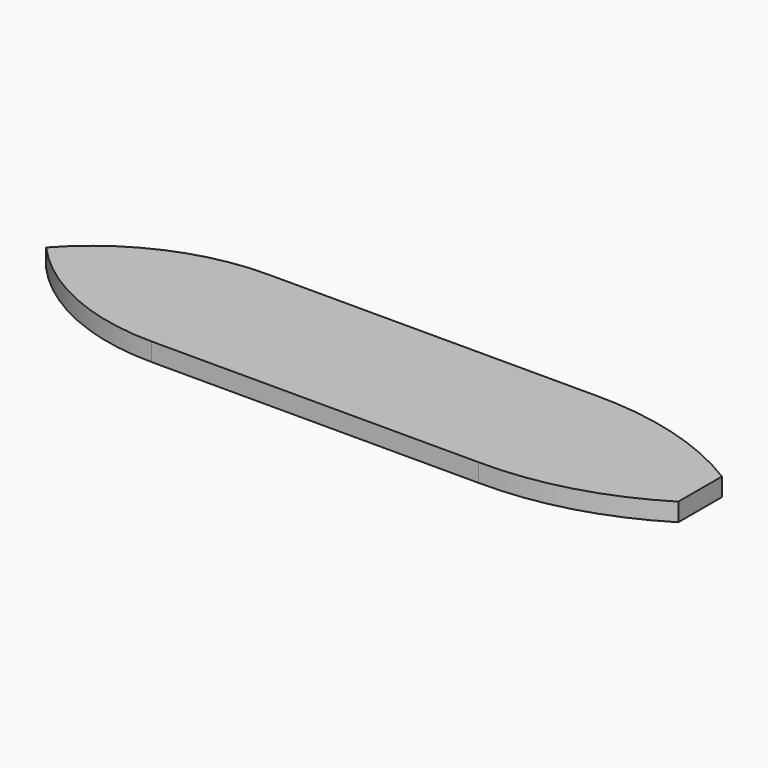
from build123d import *

# Parameters (mm, degrees)
F1_DEPTH      = 50.8
F1_DEPTH_BACK = 50.8


# Not quite as in the source:
# - the program builds the solid bodies; features that only make, move or delete a surface that nothing else refers to are left out


with BuildPart() as f1:
    # F0 (on Top) → F1 (new body, two sides)
    with BuildSketch(Plane.XY) as f1_sk:
        with BuildLine():
            Line((1828.8, -152.4), (1828.8, 152.4))
            ThreePointArc((1828.8, 152.4), (1389.7426827553, 344.713657919), (914.4, 406.4))
            Line((914.4, 406.4), (0, 406.4))
            Line((0, 406.4), (-914.4, 406.4))
            ThreePointArc((-914.4, 406.4), (-1414.7219763312, 300.2244467453), (-1828.8, 0))
            ThreePointArc((-1828.8, 0), (-1414.7219763312, -300.2244467453), (-914.4, -406.4))
            Line((-914.4, -406.4), (0, -406.4))
            Line((0, -406.4), (914.4, -406.4))
            ThreePointArc((914.4, -406.4), (1389.7426827553, -344.713657919), (1828.8, -152.4))
        make_face()
    extrude(amount=F1_DEPTH)
    extrude(f1_sk.sketch, amount=-F1_DEPTH_BACK)


solid = f1.part
